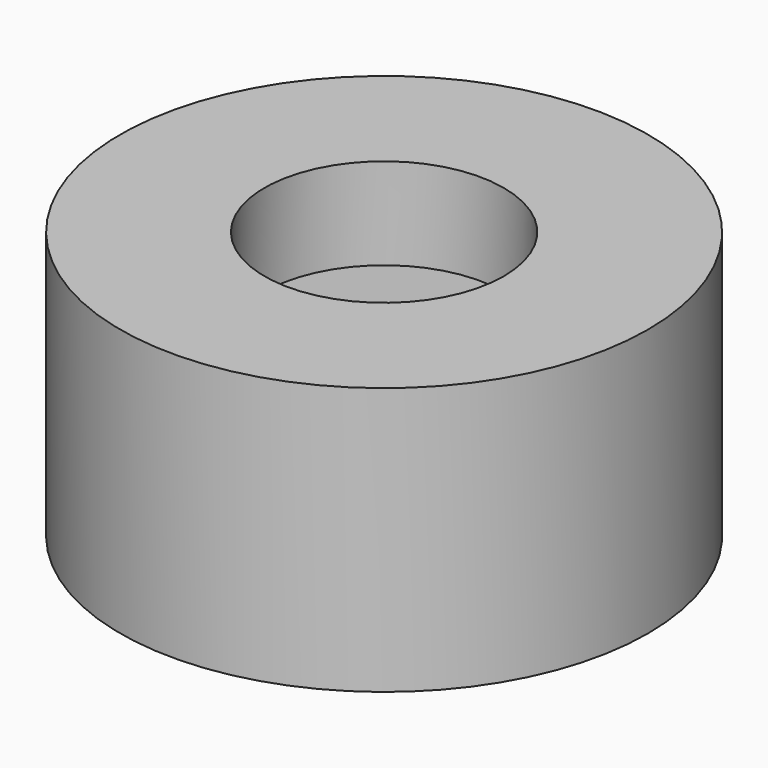
from build123d import *

# Parameters (mm, degrees)
F0_R     = 3.75
F0_R_2   = 1.7
F1_DEPTH = 3.8
F3_DEPTH = 2.5


# Not quite as in the source:
# - a feature of the source that left no trace in its solid (it failed there, or was rolled back) is left out


with BuildPart() as f1:
    # F0 (on Top) → F1 (new body)
    with BuildSketch(Plane.XY):
        with Locations((56.9799989462, -33.0372825265)):
            Circle(F0_R)
        with Locations((56.9799989462, -33.0372825265)):
            Circle(F0_R_2, mode=Mode.SUBTRACT)
    extrude(amount=F1_DEPTH)

    # F2 (on face) → F3 (cut)
    with BuildSketch(Plane(origin=(0, 0, 0), x_dir=(1, 0, 0), z_dir=(0, 0, -1))):
        Polygon((59.9799989462, 31.3052317189), (59.9799989462, 34.7693333341), (56.9799989462, 36.5013841416), (53.9799989462, 34.7693333341), (53.9799989462, 31.3052317189), (56.9799989462, 29.5731809114), align=None)
    extrude(amount=-F3_DEPTH, mode=Mode.SUBTRACT)


solid = f1.part
